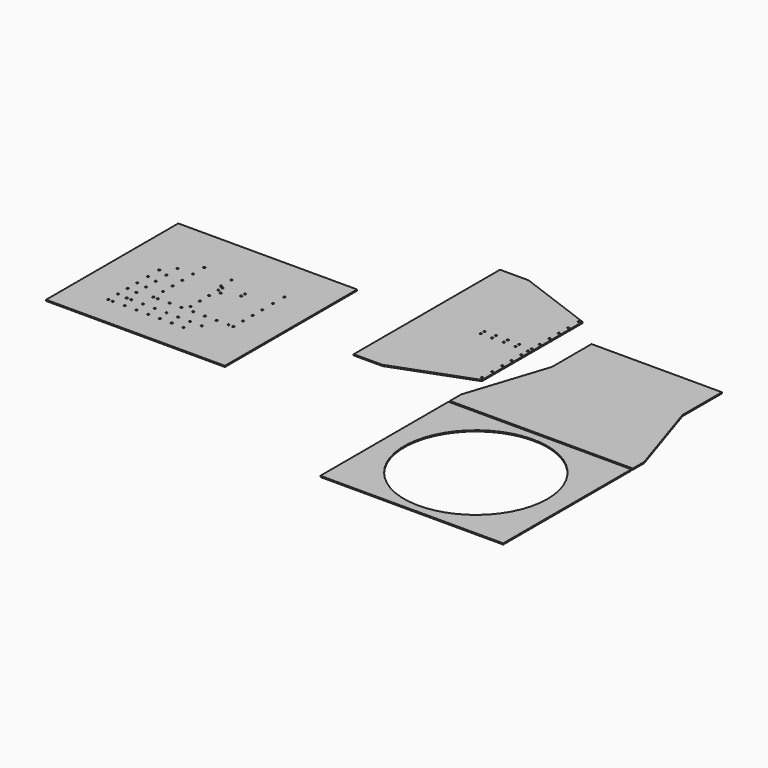
from build123d import *

# Parameters (mm, degrees)
F0_R     = 0.6291300435
F0_R_2   = 0.6332426452
F0_R_3   = 0.6321071221
F0_R_4   = 0.6831497721
F0_R_5   = 0.6652658208
F0_R_6   = 0.6497405611
F1_DEPTH = 0.762
F0_W     = 121.1580000409
F0_H     = 106.1233448563
F0_R_7   = 47.4620730635
F0_W_2   = 86.36
F0_H_2   = 32.7497554244
F0_W_3   = 118.4642314911
F0_H_3   = 109.4736345112
F0_R_8   = 0.6380048555


# Not quite as in the source:
# - ends of sketch curves that miss each other by under 0.0002 mm in the source are joined


with BuildPart() as f1:
    # F0 (on Top) → F1 (new body)
    with BuildSketch(Plane.XY):
        with BuildLine():
            Line((-23.2954401877, 99.7177349776), (-23.2954401877, 100.7407097936))
            Line((-23.2954401877, 100.7407097936), (-24.9238666147, 101.3461614512))
            Line((-24.9238666147, 101.3461614512), (-24.9238666147, 100.3674755386))
            ThreePointArc((-24.9238666147, 100.3674755386), (-24.464430658, 100.1771709343), (-24.2741260536, 99.7177349776))
            Line((-24.2741260536, 99.7177349776), (-23.295440141, 99.7177349776))
        make_face()
        with BuildLine():
            Line((-23.2954401877, 17.4287097936), (-23.2954401877, 99.7177349776))
            Line((-23.295440141, 99.7177349776), (-24.2741260536, 99.7177349776))
            ThreePointArc((-24.2741260536, 99.7177349776), (-25.3833025714, 99.2582990208), (-24.9238666147, 100.3674755386))
            Line((-24.9238666147, 100.3674755386), (-24.9238666147, 101.3461614512))
            Line((-24.9238666147, 101.3461614512), (-61.3954401877, 114.9063532467))
            Line((-61.3954401877, 114.9063532467), (-61.3954401877, 3.2630663405))
            Line((-61.3954401877, 3.2630663405), (-23.2954401877, 17.4287097936))
        make_face()
        with Locations((-24.9135376631, 19.5642051806)):
            Circle(F0_R, mode=Mode.SUBTRACT)
        with Locations((-24.9238663907, 27.9575124074)):
            Circle(F0_R_2, mode=Mode.SUBTRACT)
        with Locations((-56.1601035297, 57.4916340411)):
            Circle(F0_R_3, mode=Mode.SUBTRACT)
        with BuildLine():
            ThreePointArc((-48.5937930891, 58.1237411632), (-48.1468258406, 57.9386012823), (-47.9616859422, 57.4916340411))
            ThreePointArc((-47.9616859422, 57.4916340411), (-49.0407602881, 57.0446667999), (-48.5937930891, 58.1237411632))
        make_face(mode=Mode.SUBTRACT)
        with Locations((-40.8496819437, 57.4916340411)):
            Circle(F0_R_3, mode=Mode.SUBTRACT)
        with Locations((-24.9238663907, 36.3790051806)):
            Circle(F0_R_4, mode=Mode.SUBTRACT)
        with Locations((-24.9238672481, 43.9152853082)):
            Circle(F0_R_5, mode=Mode.SUBTRACT)
        with Locations((-24.9238672481, 52.148692377)):
            Circle(F0_R_6, mode=Mode.SUBTRACT)
        with Locations((-33.105560055, 57.4916340411)):
            Circle(F0_R_3, mode=Mode.SUBTRACT)
        with BuildLine():
            ThreePointArc((-24.2917600637, 57.49163313), (-25.3708344096, 57.0446658888), (-24.9238672105, 58.1237402522))
            ThreePointArc((-24.9238672105, 58.1237402522), (-24.4768999621, 57.9386003713), (-24.2917600637, 57.49163313))
        make_face(mode=Mode.SUBTRACT)
        with Locations((-56.1601036542, 60.6777873683)):
            Circle(F0_R_3, mode=Mode.SUBTRACT)
        with BuildLine():
            ThreePointArc((-47.9616860667, 60.6777873683), (-48.1468259476, 60.2308201445), (-48.5937931642, 60.0456802461))
            ThreePointArc((-48.5937931642, 60.0456802461), (-49.0407604301, 61.124754592), (-47.9616860667, 60.6777873683))
        make_face(mode=Mode.SUBTRACT)
        with Locations((-40.8496820682, 60.6777873683)):
            Circle(F0_R_3, mode=Mode.SUBTRACT)
        with Locations((-33.1055601795, 60.6777873683)):
            Circle(F0_R_3, mode=Mode.SUBTRACT)
        with BuildLine():
            ThreePointArc((-24.9238672857, 60.0486564137), (-25.368729439, 61.1226485686), (-24.2947372668, 60.6777864572))
            ThreePointArc((-24.2947372668, 60.6777864572), (-24.4790051816, 60.2329243459), (-24.9238672857, 60.0486564137))
        make_face(mode=Mode.SUBTRACT)
        with Locations((-24.9238672481, 67.2799982802)):
            Circle(F0_R, mode=Mode.SUBTRACT)
        with Locations((-24.9238672481, 75.4001476542)):
            Circle(F0_R, mode=Mode.SUBTRACT)
        with Locations((-24.9238672481, 83.1920728759)):
            Circle(F0_R, mode=Mode.SUBTRACT)
        with Locations((-24.9238672481, 90.8874832765)):
            Circle(F0_R, mode=Mode.SUBTRACT)
        Polygon((-61.3954401877, 3.2630663405), (-61.3954401877, 114.9063532467), (-74.1908550262, 119.6637097936), (-93.1454401877, 119.6637097337), (-93.1454401877, -1.4942902663), (-74.1908550262, -1.4942902064), align=None)
    extrude(amount=F1_DEPTH)


with BuildPart() as f1b:
    # F0 (on Top) → F1, piece 2 (new body)
    with BuildSketch(Plane.XY):
        with Locations((39.0361677242, -65.5711358995)):
            Rectangle(F0_W, F0_H)
        with Locations((39.0361677242, -65.5711358995)):
            Circle(F0_R_7, mode=Mode.SUBTRACT)
    extrude(amount=F1_DEPTH)


with BuildPart() as f1c:
    # F0 (on Top) → F1, piece 3 (new body)
    with BuildSketch(Plane.XY):
        Polygon((-21.5428358989, -1.8992669303), (-21.542834118, -11.2972669303), (99.615165882, -11.2972669303), (99.615165882, -1.8992669303), (82.216165882, 51.4898966411), (-4.143834118, 51.4898966411), align=None)
        with Locations((39.036165882, 67.8647743533)):
            Rectangle(F0_W_2, F0_H_2)
    extrude(amount=F1_DEPTH)


with BuildPart() as f1d:
    # F0 (on Top) → F1, piece 4 (new body)
    with BuildSketch(Plane.XY):
        with Locations((-196.3021159172, 1.4834981412)):
            Rectangle(F0_W_3, F0_H_3)
        with Locations((-230.4464508814, -33.0452823357)):
            Circle(F0_R_3, mode=Mode.SUBTRACT)
        with Locations((-227.4049893772, -33.0452823357)):
            Circle(F0_R_3, mode=Mode.SUBTRACT)
        with Locations((-219.6325893772, -33.0452823357)):
            Circle(F0_R_3, mode=Mode.SUBTRACT)
        with Locations((-211.8601893772, -33.0452823357)):
            Circle(F0_R_3, mode=Mode.SUBTRACT)
        with Locations((-204.0877893772, -33.0452823357)):
            Circle(F0_R_3, mode=Mode.SUBTRACT)
        with Locations((-196.3153893772, -33.0452823357)):
            Circle(F0_R_3, mode=Mode.SUBTRACT)
        with Locations((-188.4733988456, -33.0452823357)):
            Circle(F0_R_3, mode=Mode.SUBTRACT)
        with Locations((-180.6580338506, -33.0476967251)):
            Circle(F0_R_3, mode=Mode.SUBTRACT)
        with Locations((-224.1231624798, -25.7459953427)):
            Circle(F0_R_3, mode=Mode.SUBTRACT)
        with Locations((-230.4679803544, -25.0466966536)):
            Circle(F0_R_3, mode=Mode.SUBTRACT)
        with Locations((-221.0817009756, -25.7459953427)):
            Circle(F0_R_3, mode=Mode.SUBTRACT)
        with Locations((-213.3093009756, -25.7459953427)):
            Circle(F0_R_3, mode=Mode.SUBTRACT)
        with Locations((-230.4918866598, -17.0456967317)):
            Circle(F0_R_3, mode=Mode.SUBTRACT)
        with Locations((-224.1446919528, -17.7474096606)):
            Circle(F0_R_3, mode=Mode.SUBTRACT)
        with Locations((-214.0666225876, -16.2586848782)):
            Circle(F0_R_3, mode=Mode.SUBTRACT)
        with Locations((-230.5157929659, -9.0446965769)):
            Circle(F0_R_3, mode=Mode.SUBTRACT)
        with Locations((-224.1685982582, -9.7464097387)):
            Circle(F0_R_3, mode=Mode.SUBTRACT)
        with Locations((-214.0881520606, -8.2600991961)):
            Circle(F0_R_3, mode=Mode.SUBTRACT)
        with Locations((-230.5424094321, -0.1366557553)):
            Circle(F0_R_3, mode=Mode.SUBTRACT)
        with Locations((-224.1925045643, -1.7454095839)):
            Circle(F0_R_3, mode=Mode.SUBTRACT)
        with Locations((-214.112058366, -0.2590992742)):
            Circle(F0_R_3, mode=Mode.SUBTRACT)
        with Locations((-205.5369009756, -25.7459953427)):
            Circle(F0_R_3, mode=Mode.SUBTRACT)
        with Locations((-197.7645009756, -25.7459953427)):
            Circle(F0_R_3, mode=Mode.SUBTRACT)
        with Locations((-189.9921009756, -25.7459953427)):
            Circle(F0_R_3, mode=Mode.SUBTRACT)
        with Locations((-211.0251610834, -16.2586848782)):
            Circle(F0_R_3, mode=Mode.SUBTRACT)
        with Locations((-203.2527610834, -16.2586848782)):
            Circle(F0_R_3, mode=Mode.SUBTRACT)
        with Locations((-195.4803610834, -16.2586848782)):
            Circle(F0_R_3, mode=Mode.SUBTRACT)
        with Locations((-182.150110444, -25.7459953427)):
            Circle(F0_R_3, mode=Mode.SUBTRACT)
        with Locations((-174.334745449, -25.7484097322)):
            Circle(F0_R_3, mode=Mode.SUBTRACT)
        with Locations((-187.7079610834, -16.2586848782)):
            Circle(F0_R_3, mode=Mode.SUBTRACT)
        with Locations((-179.9355610834, -16.2586848782)):
            Circle(F0_R_3, mode=Mode.SUBTRACT)
        with Locations((-172.0935705518, -16.2586848782)):
            Circle(F0_R_3, mode=Mode.SUBTRACT)
        with Locations((-192.3992521438, -12.5447819406)):
            Circle(F0_R_3, mode=Mode.SUBTRACT)
        with Locations((-192.3992521438, -4.7723819406)):
            Circle(F0_R_3, mode=Mode.SUBTRACT)
        with Locations((-164.2782055568, -16.2610992677)):
            Circle(F0_R_3, mode=Mode.SUBTRACT)
        with Locations((-161.0920522296, -16.2610992677)):
            Circle(F0_R_8, mode=Mode.SUBTRACT)
        with Locations((-161.0920404233, -8.2600992677)):
            Circle(F0_R_8, mode=Mode.SUBTRACT)
        with Locations((-161.0920404233, -0.2590992677)):
            Circle(F0_R_3, mode=Mode.SUBTRACT)
        with Locations((-224.2191210306, 7.1626312376)):
            Circle(F0_R_3, mode=Mode.SUBTRACT)
        with Locations((-214.1359646721, 7.7419008806)):
            Circle(F0_R_3, mode=Mode.SUBTRACT)
        with Locations((-230.5704598746, 9.2513104901)):
            Circle(F0_R_3, mode=Mode.SUBTRACT)
        with Locations((-224.2471714731, 16.550597483)):
            Circle(F0_R_3, mode=Mode.SUBTRACT)
        with Locations((-214.1625811384, 16.6499417021)):
            Circle(F0_R_3, mode=Mode.SUBTRACT)
        with Locations((-214.1906315809, 26.0379079475)):
            Circle(F0_R_3, mode=Mode.SUBTRACT)
        with Locations((-192.538488594, 3.0000180594)):
            Circle(F0_R_3, mode=Mode.SUBTRACT)
        with Locations((-189.6270393959, 8.9803204777)):
            Circle(F0_R_3, mode=Mode.SUBTRACT)
        with Locations((-192.538488594, 10.7724180594)):
            Circle(F0_R_3, mode=Mode.SUBTRACT)
        with Locations((-194.5303856338, 15.2733816274)):
            Circle(F0_R_3, mode=Mode.SUBTRACT)
        with Locations((-192.538488594, 13.9673350528)):
            Circle(F0_R_3, mode=Mode.SUBTRACT)
        with Locations((-179.2514622211, 12.9540003836)):
            Circle(F0_R_3, mode=Mode.SUBTRACT)
        with Locations((-194.5303855871, 24.0041953553)):
            Circle(F0_R_3, mode=Mode.SUBTRACT)
        with Locations((-179.2514623457, 16.1401537108)):
            Circle(F0_R_3, mode=Mode.SUBTRACT)
        with Locations((-161.0920404233, 7.7419007323)):
            Circle(F0_R_3, mode=Mode.SUBTRACT)
        with Locations((-161.0920404233, 16.6499411538)):
            Circle(F0_R_3, mode=Mode.SUBTRACT)
        with Locations((-161.0920404233, 26.0379075528)):
            Circle(F0_R_3, mode=Mode.SUBTRACT)
    extrude(amount=F1_DEPTH)


solid = Compound([f1.part, f1b.part, f1c.part, f1d.part])
